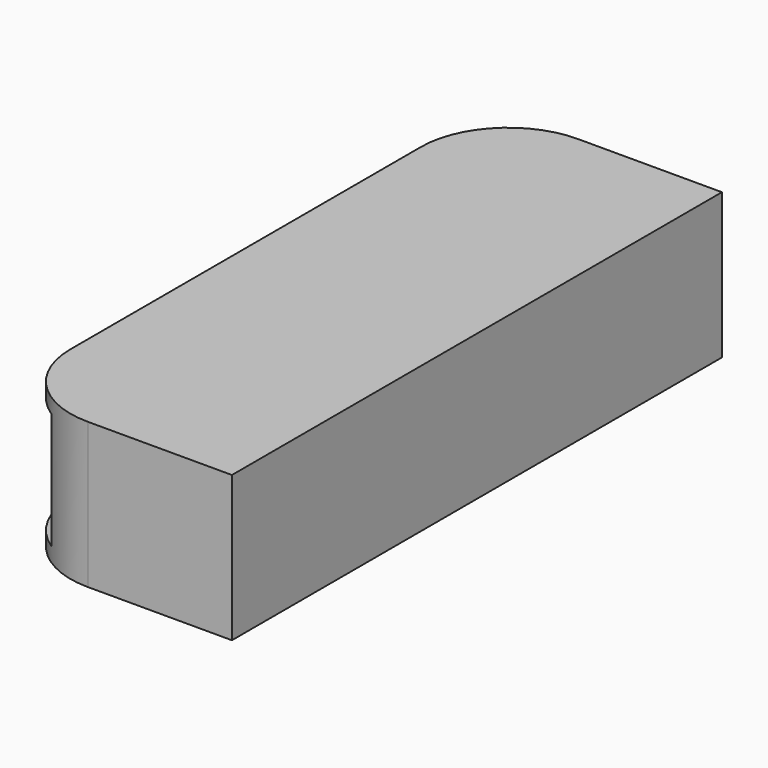
from build123d import *

# Parameters (mm, degrees)
F0_W        = 39.7482234985
F0_H        = 105.248818174
F1_DEPTH    = 25
F2_T        = -2.5
F3_T1_DEPTH = 100


# Not quite as in the source:
# - a fillet or chamfer that OpenCascade refuses, or shapes differently, is made with other operations: its cross-section is extruded or revolved along the edge and cut away or added


with BuildPart() as f1:
    # F0 (on Top) → F1 (new body)
    with BuildSketch(Plane.XY):
        with Locations((1.5861960128, 22.0201415941)):
            Rectangle(F0_W, F0_H)
    extrude(amount=F1_DEPTH)

    # F2
    f2_openings = [f1.faces().sort_by_distance(p)[0] for p in [
        (-18.287916, 22.020142, 12.5),
    ]]
    offset(amount=F2_T, openings=f2_openings)

    # F3: fillet of radius 15 on 2 edges, made by hand

    # F3_s2 → F3_t1 (cut)
    with BuildSketch(Plane.XY.offset(-37.5)):
        with BuildLine():
            ThreePointArc((-3.2879157364, 74.6445506811), (-13.8945174542, 70.2511523989), (-18.2879157364, 59.6445506811))
            Line((-18.2879157364, 59.6445506811), (-18.2879157364, 74.6445506811))
            Line((-18.2879157364, 74.6445506811), (-3.2879157364, 74.6445506811))
        make_face()
        with BuildLine():
            ThreePointArc((-3.2879157364, -30.6042674929), (-13.8945174542, -26.2108692107), (-18.2879157364, -15.6042674929))
            Line((-18.2879157364, -15.6042674929), (-18.2879157364, -30.6042674929))
            Line((-18.2879157364, -30.6042674929), (-3.2879157364, -30.6042674929))
        make_face()
    extrude(amount=F3_T1_DEPTH, mode=Mode.SUBTRACT)


solid = f1.part
